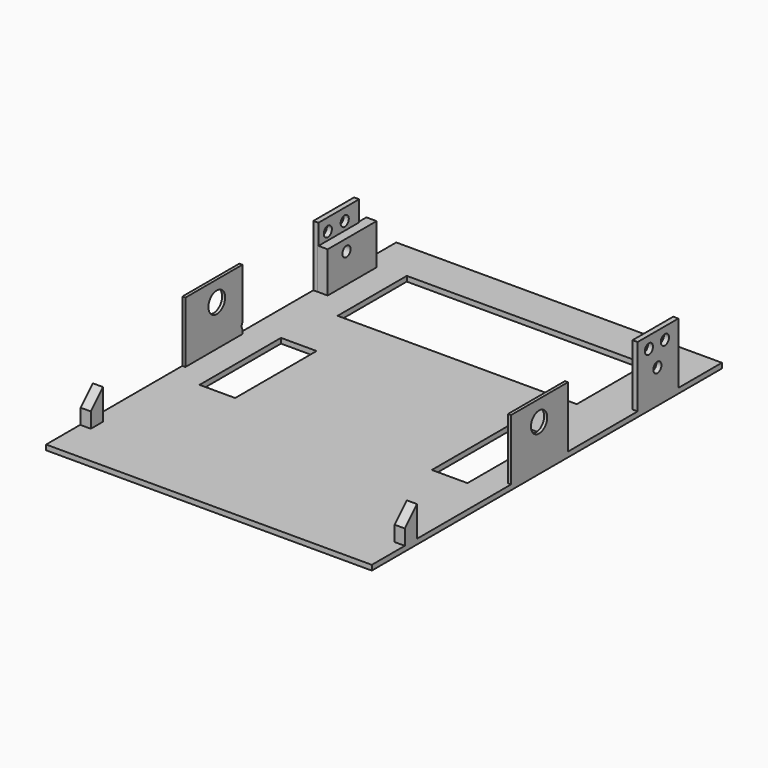
from build123d import *

# Parameters (mm, degrees)
F0_W      = 320
F0_H      = 430
F1_DEPTH  = 5
F2_W      = 35
F2_H      = 100
F3_DEPTH  = 5
F4_W      = 35
F4_H      = 100
F5_DEPTH  = 5
F7_DEPTH  = 5
F8_W      = 3
F8_H      = 70
F9_DEPTH  = 60
F10_W     = 3
F10_H     = 70
F11_DEPTH = 60
F12_W     = 5
F12_H     = 50
F13_DEPTH = 60
F14_W     = 5
F14_H     = 50
F15_DEPTH = 60
F16_R     = 10
F17_DEPTH = 120
F18_R     = 10.2640382995
F19_DEPTH = 240
F20_W     = 10
F20_H     = 15
F21_DEPTH = 30
F22_SIZE  = 14.99999
F23_W     = 10
F23_H     = 15
F24_DEPTH = 30
F25_SIZE  = 14.99999
F26_W     = 10
F26_H     = 60
F27_DEPTH = 40
F28_R     = 5
F29_DEPTH = 240
F30_R     = 5
F31_DEPTH = 240
F32_R     = 5
F33_DEPTH = 250
F34_R     = 5
F35_DEPTH = 300
F36_R     = 5
F37_DEPTH = 300
F38_R     = 5
F39_DEPTH = 300
F40_R     = 10
F41_DEPTH = 207.2868810425
F42_R     = 5
F43_DEPTH = 207.2868810425
F44_R     = 5
F45_DEPTH = 207.2868810425
F46_R     = 5
F47_DEPTH = 207.2868810425
F48_R     = 5
F49_DEPTH = 207.2868810425


# Not quite as in the source:
# - a fillet or chamfer is up to 0.001 mm smaller than in the source, because OpenCascade refuses the exact size


with BuildPart() as f1:
    # F0 (on Top) → F1 (new body)
    with BuildSketch(Plane.XY):
        with Locations((-47.2858810425, 185.3322760761)):
            Rectangle(F0_W, F0_H)
    extrude(amount=F1_DEPTH)

    # F2 (on face) → F3 (cut)
    with BuildSketch(Plane.XY.offset(5)):
        with Locations((-159.7858810425, 171.3026314974)):
            Rectangle(F2_W, F2_H)
    extrude(amount=-F3_DEPTH, mode=Mode.SUBTRACT)

    # F4 (on face) → F5 (cut)
    with BuildSketch(Plane(origin=(0, 0, 0), x_dir=(1, 0, 0), z_dir=(0, 0, -1))):
        with Locations((67.7159577608, -172.2117364407)):
            Rectangle(F4_W, F4_H)
    extrude(amount=-F5_DEPTH, mode=Mode.SUBTRACT)

    # F6 (on face) → F7 (cut)
    with BuildSketch(Plane.XY.offset(5)):
        Polygon((68.7382593751, 362.0384633541), (-166.2617406249, 362.0384633541), (-166.2617406249, 277.0384633541), (-65.0134384632, 277.0384633541), (-48.7617406249, 277.0384633541), (68.7382593751, 277.0384633541), align=None)
    extrude(amount=-F7_DEPTH, mode=Mode.SUBTRACT)

    # F8 (on face) → F9 (join)
    with BuildSketch(Plane.XY.offset(5)):
        with Locations((-205.7858810425, 172.665733695)):
            Rectangle(F8_W, F8_H)
    extrude(amount=F9_DEPTH)

    # F10 (on face) → F11 (join)
    with BuildSketch(Plane.XY.offset(5)):
        with Locations((111.2141189575, 176.3021534681)):
            Rectangle(F10_W, F10_H)
    extrude(amount=F11_DEPTH)

    # F12 (on face) → F13 (join)
    with BuildSketch(Plane.XY.offset(5)):
        with Locations((-204.7858810425, 323.5781848431)):
            Rectangle(F12_W, F12_H)
    extrude(amount=F13_DEPTH)

    # F14 (on face) → F15 (join)
    with BuildSketch(Plane.XY.offset(5)):
        with Locations((110.2141189575, 321.7600047588)):
            Rectangle(F14_W, F14_H)
    extrude(amount=F15_DEPTH)

    # F16 (on Right) → F17 (cut)
    with BuildSketch(Plane.YZ):
        with Locations((175.784942263, 45.0581042336)):
            Circle(F16_R)
    extrude(amount=F17_DEPTH, mode=Mode.SUBTRACT)

    # F18 (on Right) → F19 (cut)
    with BuildSketch(Plane.YZ):
        with Locations((176.2254685163, 45.2939495444)):
            Circle(F18_R)
    extrude(amount=-F19_DEPTH, mode=Mode.SUBTRACT)

    # F20 (on face) → F21 (join)
    with BuildSketch(Plane.XY.offset(5)):
        with Locations((107.7141189575, 18.3457679302)):
            Rectangle(F20_W, F20_H)
    extrude(amount=F21_DEPTH)

    # F22 (size 15 in the source; OpenCascade refuses exactly that, so slightly less here)
    f22_edges = [f1.edges().sort_by_distance(p)[0] for p in [
        (107.714119, 10.845768, 35),
    ]]
    chamfer(f22_edges, length=F22_SIZE)

    # F23 (on face) → F24 (join)
    with BuildSketch(Plane.XY.offset(5)):
        with Locations((-201.83388412, 19.7091826051)):
            Rectangle(F23_W, F23_H)
    extrude(amount=F24_DEPTH)

    # F25 (size 15 in the source; OpenCascade refuses exactly that, so slightly less here)
    f25_edges = [f1.edges().sort_by_distance(p)[0] for p in [
        (-201.833884, 12.209183, 35),
    ]]
    chamfer(f25_edges, length=F25_SIZE)

    # F26 (on face) → F27 (join)
    with BuildSketch(Plane.XY.offset(5)):
        with Locations((-198.1973099709, 328.5773980618)):
            Rectangle(F26_W, F26_H)
    extrude(amount=F27_DEPTH)

    # F28 (on Right) → F29 (cut)
    with BuildSketch(Plane.YZ):
        with Locations((310.6648027897, 53.3718466759)):
            Circle(F28_R)
    extrude(amount=F29_DEPTH, mode=Mode.SUBTRACT)

    # F30 (on Right) → F31 (cut)
    with BuildSketch(Plane.YZ):
        with Locations((330.2825987339, 53.3718466759)):
            Circle(F30_R)
    extrude(amount=F31_DEPTH, mode=Mode.SUBTRACT)

    # F32 (on Right) → F33 (cut)
    with BuildSketch(Plane.YZ):
        with Locations((321.0507035255, 33.1770926714)):
            Circle(F32_R)
    extrude(amount=F33_DEPTH, mode=Mode.SUBTRACT)

    # F34 (on Right) → F35 (cut)
    with BuildSketch(Plane.YZ):
        with Locations((310.0878298283, 52.794855088)):
            Circle(F34_R)
    extrude(amount=-F35_DEPTH, mode=Mode.SUBTRACT)

    # F36 (on Right) → F37 (cut)
    with BuildSketch(Plane.YZ):
        with Locations((330.8595716953, 53.3718466759)):
            Circle(F36_R)
    extrude(amount=-F37_DEPTH, mode=Mode.SUBTRACT)

    # F38 (on Right) → F39 (cut)
    with BuildSketch(Plane.YZ):
        with Locations((321.627676487, 33.7540879846)):
            Circle(F38_R)
    extrude(amount=-F39_DEPTH, mode=Mode.SUBTRACT)

    # F40 (on Right) → F41 (cut, through all)
    with BuildSketch(Plane.YZ):
        with Locations((228.0015647411, 27.0902961493)):
            Circle(F40_R)
    extrude(amount=-F41_DEPTH, mode=Mode.SUBTRACT)

    # F42 (on Right) → F43 (cut, through all)
    with BuildSketch(Plane.YZ):
        with Locations((241.425678134, 41.8319888413)):
            Circle(F42_R)
    extrude(amount=-F43_DEPTH, mode=Mode.SUBTRACT)

    # F44 (on Right) → F45 (cut, through all)
    with BuildSketch(Plane.YZ):
        with Locations((240.8486753702, 12.9823405296)):
            Circle(F44_R)
    extrude(amount=-F45_DEPTH, mode=Mode.SUBTRACT)

    # F46 (on Right) → F47 (cut, through all)
    with BuildSketch(Plane.YZ):
        with Locations((213.0800783634, 41.6209772229)):
            Circle(F46_R)
    extrude(amount=-F47_DEPTH, mode=Mode.SUBTRACT)

    # F48 (on Right) → F49 (cut, through all)
    with BuildSketch(Plane.YZ):
        with Locations((211.7366492748, 12.104251422)):
            Circle(F48_R)
    extrude(amount=-F49_DEPTH, mode=Mode.SUBTRACT)


solid = f1.part
